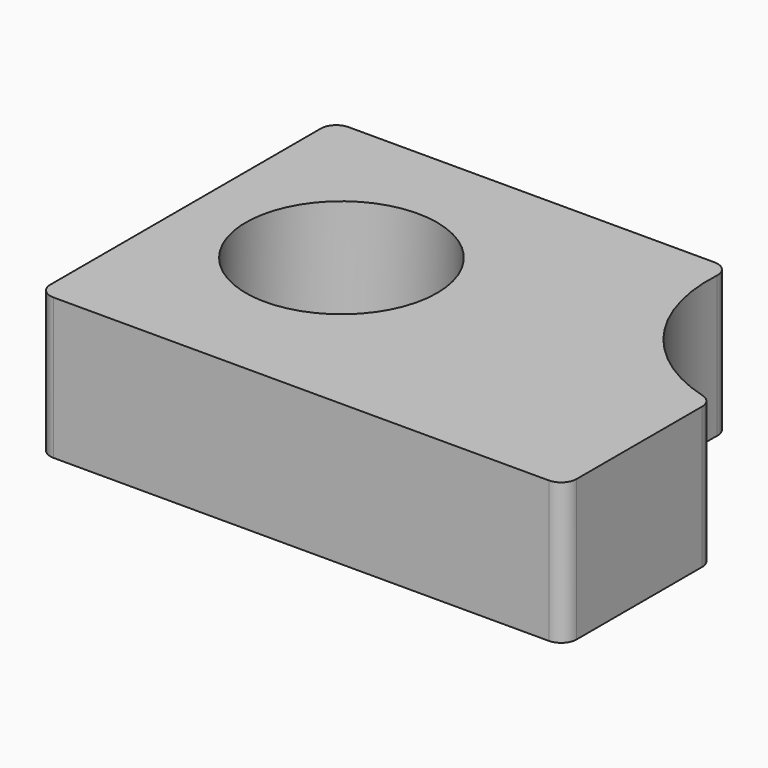
from build123d import *

# Parameters (mm, degrees)
F0_W        = 186.2502396107
F0_H        = 130.5641233921
F1_DEPTH    = 50
F2_R        = 33.843412588
F3_DEPTH    = 153
F5_DEPTH    = 98
F6_T        = -2.5
F7_DEPTH    = 34.7
F8_T1_DEPTH = 77.2897189396
F8_T3_DEPTH = 80.4969668156
F8_T5_DEPTH = 71.5460241694


# Not quite as in the source:
# - a fillet or chamfer that OpenCascade refuses, or shapes differently, is made with other operations: its cross-section is extruded or revolved along the edge and cut away or added


with BuildPart() as f1:
    # F0 (on Top) → F1 (new body)
    with BuildSketch(Plane.XY):
        with Locations((-4.4038519263, -2.9969513416)):
            Rectangle(F0_W, F0_H)
    extrude(amount=F1_DEPTH)

    # F2 (on face) → F3 (cut)
    with BuildSketch(Plane(origin=(0, 0, 0), x_dir=(1, 0, 0), z_dir=(0, 0, -1))):
        with Locations((-44.7623804212, 0)):
            Circle(F2_R)
    extrude(amount=-F3_DEPTH, mode=Mode.SUBTRACT)

    # F4 (on face) → F5 (cut)
    with BuildSketch(Plane.XY.offset(50)):
        with BuildLine():
            Line((88.721267879, 62.2851103544), (43.5578748584, 62.2851103544))
            ThreePointArc((43.5578748584, 62.2851103544), (52.9449353899, 20.5157751148), (88.721267879, -2.9969513416))
            Line((88.721267879, -2.9969513416), (88.721267879, 62.2851103544))
        make_face()
    extrude(amount=-F5_DEPTH, mode=Mode.SUBTRACT)

    # F6
    f6_openings = [f1.faces().sort_by_distance(p)[0] for p in [
        (-26.985548, 62.28511, 25),
    ]]
    offset(amount=F6_T, openings=f6_openings)

    # F7 (add): a face of the model
    f7_faces = [f1.faces().sort_by_distance(p)[0] for p in [
        (-5.8734353471, -8.457374128, 50),
    ]]
    extrude(f7_faces, amount=-F7_DEPTH)

    # F8: fillet of radius 5.4579437879 on 5 edges, made by hand

    # F8_s2 → F8_t1 (cut)
    with BuildSketch(Plane.XY.offset(-13.6448594698)):
        with BuildLine():
            ThreePointArc((-97.5289717317, -62.8210692498), (-95.9303770075, -66.6804183135), (-92.0710279438, -68.2790130377))
            Line((-92.0710279438, -68.2790130377), (-97.5289717317, -68.2790130377))
            Line((-97.5289717317, -68.2790130377), (-97.5289717317, -62.8210692498))
        make_face()
        with BuildLine():
            ThreePointArc((83.2633240911, -68.2790130377), (87.1226731549, -66.6804183135), (88.721267879, -62.8210692498))
            Line((88.721267879, -62.8210692498), (88.721267879, -68.2790130377))
            Line((88.721267879, -68.2790130377), (83.2633240911, -68.2790130377))
        make_face()
        with BuildLine():
            ThreePointArc((-92.0710279438, 62.2851103544), (-95.9303770075, 60.6865156303), (-97.5289717317, 56.8271665665))
            Line((-97.5289717317, 56.8271665665), (-97.5289717317, 62.2851103544))
            Line((-97.5289717317, 62.2851103544), (-92.0710279438, 62.2851103544))
        make_face()
    extrude(amount=F8_T1_DEPTH, mode=Mode.SUBTRACT)

    # F8_s4 → F8_t3 (cut)
    with BuildSketch(Plane.XY.offset(-15.2484834078)):
        with BuildLine():
            ThreePointArc((37.4584814953, 62.2851103544), (41.4337624229, 60.5669916879), (42.9062677149, 56.4943367342))
            ThreePointArc((42.9062677149, 56.4943367342), (43.1581721547, 59.3980390485), (43.5578748584, 62.2851103544))
            Line((43.5578748584, 62.2851103544), (37.4584814953, 62.2851103544))
        make_face()
    extrude(amount=F8_T3_DEPTH, mode=Mode.SUBTRACT)

    # F8_s6 → F8_t5 (cut)
    with BuildSketch(Plane.XY.offset(-10.7730120847)):
        with BuildLine():
            ThreePointArc((88.721267879, -7.3061561755), (87.605956573, -3.99999624), (84.7158424133, -2.0450402373))
            ThreePointArc((84.7158424133, -2.0450402373), (86.7099755288, -2.557096868), (88.721267879, -2.9969513416))
            Line((88.721267879, -2.9969513416), (88.721267879, -7.3061561755))
        make_face()
    extrude(amount=F8_T5_DEPTH, mode=Mode.SUBTRACT)


solid = f1.part
